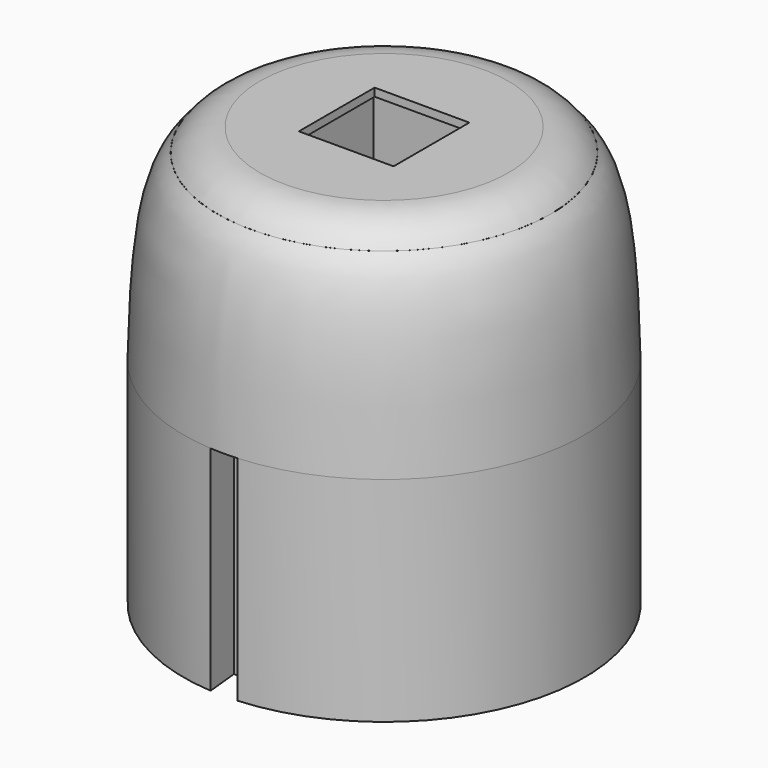
from build123d import *

# Parameters (mm, degrees)
F2_R      = 62.5
F2_W      = 38.8455463488
F2_H      = 38.8455463488
F3_DEPTH  = 157.39
F8_W      = 38.8455463488
F8_H      = 38.8455463488
F8_W_2    = 35.5
F8_H_2    = 35.5
F9_DEPTH  = 3
F11_DEPTH = 80
F12_R     = 6.35
F13_DEPTH = 12.7


# Not quite as in the source:
# - a feature names something its author has since deleted; it is built from what else it names


with BuildPart() as f1:
    # F0 (on Front) → F1 (revolve)
    with BuildSketch(Plane.XZ):
        with BuildLine():
            ThreePointArc((-62.42, 0), (-60.0517541619, 76.462422463), (-50.8, 152.4))
            Line((-50.8, 152.4), (-45.72, 152.4))
            Line((-45.72, 152.4), (-45.72, 157.4))
            add(Edge.make_bspline(
                [(-75.12, 80), (-74.447497537, 106.2833289956), (-73.373072159, 148.2749606206), (-53.2483071241, 154.9157878093), (-45.72, 157.4)],
                knots=[0, 0, 0, 0, 0.6259182599, 1, 1, 1, 1], degree=3))
            Line((-75.12, 80), (-75.12, 0))
            Line((-75.12, 0), (-62.42, 0))
        make_face()
    revolve(axis=Axis((0, 0, 76.2), (0, 0, 1)))

    # F2 (on Top) → F3 (join)
    with BuildSketch(Plane.XY):
        Circle(F2_R)
        Rectangle(F2_W, F2_H, mode=Mode.SUBTRACT)
    extrude(amount=F3_DEPTH)

    # F5 (on Front) → F6 (revolve, cut)
    with BuildSketch(Plane.XZ):
        with BuildLine():
            Line((-19.432, 0), (0, 0))
            Line((0, 0), (0, 117.132))
            Line((0, 117.132), (-19.432, 117.132))
            add(Edge.make_bspline(
                [(-49.6, 0), (-46.3600523587, 18.5581395922), (-40.1579876774, 54.0830291461), (-27.905682613, 101.3967550255), (-21.7260374714, 112.8720762759), (-19.432, 117.132)],
                knots=[0, 0, 0, 0, 0.4074955134, 0.7800476463, 1, 1, 1, 1], degree=3))
            Line((-49.6, 0), (-19.432, 0))
        make_face()
    revolve(axis=Axis((0, 0, 58.566), (0, 0, -1)), mode=Mode.SUBTRACT)

    # F4 (on Front) → F7 (revolve, cut)
    with BuildSketch(Plane.XZ):
        with BuildLine():
            Line((-59.5792606473, 163.4935438633), (-68.9641386271, 155.4379612207))
            Line((-68.9641386271, 155.4379612207), (-62.5000447035, 148.8302797079))
            ThreePointArc((-62.5000447035, 148.8302797079), (-55.5803045517, 155.0029325492), (-46.5795062482, 157.2322994471))
            Line((-46.5795062482, 157.2322994471), (0, 157.2322994471))
            Line((0, 157.2322994471), (0, 165.5570715666))
            Line((0, 165.5570715666), (-59.5792606473, 163.4935438633))
        make_face()
    revolve(axis=Axis((0, 0, 161.3946855068), (0, 0, 1)), mode=Mode.SUBTRACT)

    # F8 (on face) → F9 (join)
    with BuildSketch(Plane.XY.offset(157.2322994471)):
        Rectangle(F8_W, F8_H)
        Rectangle(F8_W_2, F8_H_2, mode=Mode.SUBTRACT)
    extrude(amount=-F9_DEPTH)

    # F10 (on face) → F11 (cut)
    with BuildSketch(Plane(origin=(0, 0, 0), x_dir=(1, 0, 0), z_dir=(0, 0, -1))):
        with BuildLine():
            Line((-6.35, 62.42), (6.35, 62.42))
            Line((6.35, 62.42), (5.08, 74.9480353312))
            ThreePointArc((5.08, 74.9480353312), (0, 75.12), (-5.08, 74.9480353312))
            Line((-5.08, 74.9480353312), (-6.35, 62.42))
        make_face()
        with BuildLine():
            ThreePointArc((-5.08, 74.9480353312), (0, 75.12), (5.08, 74.9480353312))
            ThreePointArc((5.08, 74.9480353312), (0, 79.5390976959), (-5.08, 74.9480353312))
        make_face()
        with BuildLine():
            Line((-6.35, -62.42), (-5.08, -74.9480353312))
            ThreePointArc((-5.08, -74.9480353312), (0, -75.12), (5.08, -74.9480353312))
            Line((5.08, -74.9480353312), (6.35, -62.42))
            Line((6.35, -62.42), (-6.35, -62.42))
        make_face()
        with BuildLine():
            ThreePointArc((5.08, -74.9480353312), (0, -75.12), (-5.08, -74.9480353312))
            ThreePointArc((-5.08, -74.9480353312), (0, -79.5390976959), (5.08, -74.9480353312))
        make_face()
    extrude(amount=-F11_DEPTH, mode=Mode.SUBTRACT)

    # F12 (on face) → F13 (cut)
    with BuildSketch(Plane(origin=(0, 0, 0), x_dir=(1, 0, 0), z_dir=(0, 0, -1))):
        with Locations((-44.1376052817, 44.1376052817)):
            Circle(F12_R)
        with Locations((44.1376052817, 44.1376052817)):
            Circle(F12_R)
        with Locations((44.1376052817, -44.1376052817)):
            Circle(F12_R)
        with Locations((-44.1376052817, -44.1376052817)):
            Circle(F12_R)
    extrude(amount=-F13_DEPTH, mode=Mode.SUBTRACT)


solid = f1.part
